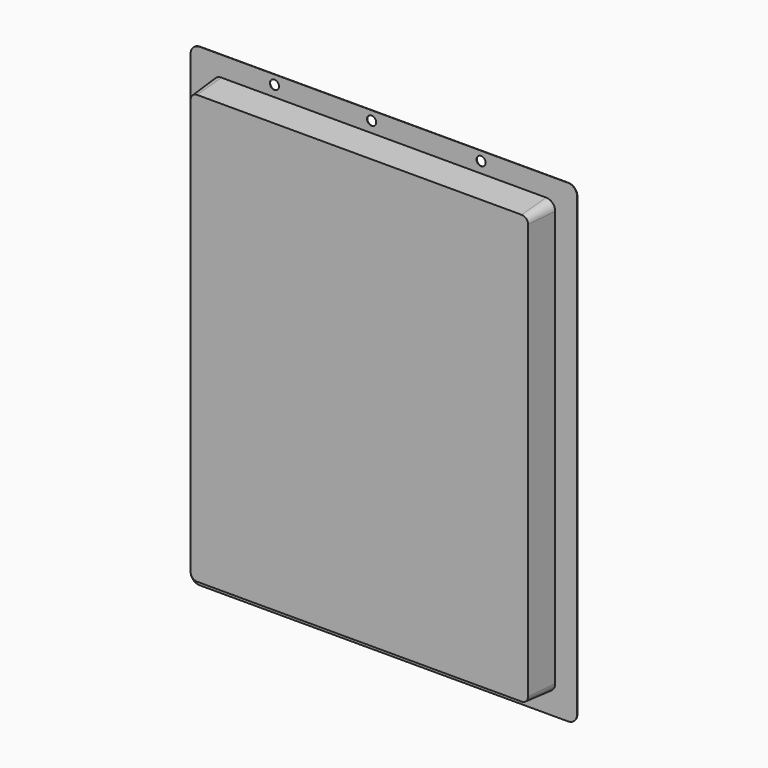
from build123d import *

# Parameters (mm, degrees)
F0_R     = 3.175
F1_DEPTH = 0.254
F2_DEPTH = 21.59
F2_TAPER = 5


# Not quite as in the source:
# - a feature names something its author has since deleted; it is built from what else it names


with BuildPart() as f1:
    # F0 (on Front) → F1 (new body)
    with BuildSketch(Plane.XZ):
        with BuildLine():
            Line((-128.27, -165.1), (128.27, -165.1))
            ThreePointArc((128.27, -165.1), (132.7601280605, -163.2401280605), (134.62, -158.75))
            Line((134.62, -158.75), (134.62, 158.75))
            ThreePointArc((134.62, 158.75), (132.7601280605, 163.2401280605), (128.27, 165.1))
            Line((128.27, 165.1), (-128.27, 165.1))
            ThreePointArc((-128.27, 165.1), (-132.7601280605, 163.2401280605), (-134.62, 158.75))
            Line((-134.62, 158.75), (-134.62, -158.75))
            ThreePointArc((-134.62, -158.75), (-132.7601280605, -163.2401280605), (-128.27, -165.1))
        make_face()
        with Locations((-76.2, -160.02)):
            Circle(F0_R, mode=Mode.SUBTRACT)
        with Locations((0, -160.02)):
            Circle(F0_R, mode=Mode.SUBTRACT)
        with Locations((78.74, -160.02)):
            Circle(F0_R, mode=Mode.SUBTRACT)
        with Locations((-76.2, 158.75)):
            Circle(F0_R, mode=Mode.SUBTRACT)
        with Locations((-8.5018249229, 158.75)):
            Circle(F0_R, mode=Mode.SUBTRACT)
        with BuildLine():
            ThreePointArc((119.38, -144.78), (117.5201280605, -149.2701280605), (113.03, -151.13))
            Line((113.03, -151.13), (76.2, -151.13))
            Line((76.2, -151.13), (-76.2, -151.13))
            Line((-76.2, -151.13), (-113.03, -151.13))
            ThreePointArc((-113.03, -151.13), (-117.5201280605, -149.2701280605), (-119.38, -144.78))
            Line((-119.38, -144.78), (-119.38, 144.78))
            ThreePointArc((-119.38, 144.78), (-117.5201280605, 149.2701280605), (-113.03, 151.13))
            Line((-113.03, 151.13), (-76.2, 151.13))
            Line((-76.2, 151.13), (76.2, 151.13))
            Line((76.2, 151.13), (113.03, 151.13))
            ThreePointArc((113.03, 151.13), (117.5201280605, 149.2701280605), (119.38, 144.78))
            Line((119.38, 144.78), (119.38, -144.78))
        make_face(mode=Mode.SUBTRACT)
        with Locations((67.6981750771, 158.75)):
            Circle(F0_R, mode=Mode.SUBTRACT)
        with BuildLine():
            Line((76.2, -151.13), (113.03, -151.13))
            ThreePointArc((113.03, -151.13), (117.5201280605, -149.2701280605), (119.38, -144.78))
            Line((119.38, -144.78), (119.38, 144.78))
            ThreePointArc((119.38, 144.78), (117.5201280605, 149.2701280605), (113.03, 151.13))
            Line((113.03, 151.13), (76.2, 151.13))
            Line((76.2, 151.13), (-76.2, 151.13))
            Line((-76.2, 151.13), (-113.03, 151.13))
            ThreePointArc((-113.03, 151.13), (-117.5201280605, 149.2701280605), (-119.38, 144.78))
            Line((-119.38, 144.78), (-119.38, -144.78))
            ThreePointArc((-119.38, -144.78), (-117.5201280605, -149.2701280605), (-113.03, -151.13))
            Line((-113.03, -151.13), (-76.2, -151.13))
            Line((-76.2, -151.13), (76.2, -151.13))
        make_face()
    extrude(amount=F1_DEPTH)

    # F0 (on Front) → F2 (join)
    with BuildSketch(Plane.XZ):
        with BuildLine():
            Line((76.2, -151.13), (113.03, -151.13))
            ThreePointArc((113.03, -151.13), (117.5201280605, -149.2701280605), (119.38, -144.78))
            Line((119.38, -144.78), (119.38, 144.78))
            ThreePointArc((119.38, 144.78), (117.5201280605, 149.2701280605), (113.03, 151.13))
            Line((113.03, 151.13), (76.2, 151.13))
            Line((76.2, 151.13), (-76.2, 151.13))
            Line((-76.2, 151.13), (-113.03, 151.13))
            ThreePointArc((-113.03, 151.13), (-117.5201280605, 149.2701280605), (-119.38, 144.78))
            Line((-119.38, 144.78), (-119.38, -144.78))
            ThreePointArc((-119.38, -144.78), (-117.5201280605, -149.2701280605), (-113.03, -151.13))
            Line((-113.03, -151.13), (-76.2, -151.13))
            Line((-76.2, -151.13), (76.2, -151.13))
        make_face()
    extrude(amount=F2_DEPTH, taper=F2_TAPER)


solid = f1.part
